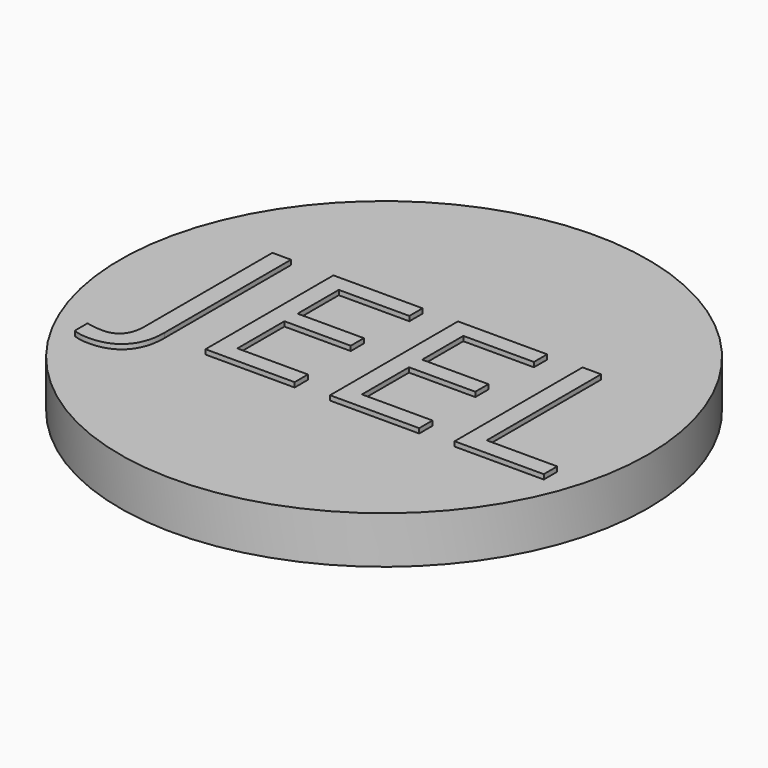
from build123d import *

# Parameters (mm, degrees)
F0_R         = 14.199997
F1_DEPTH     = 2.54
F2_TEXT_SIZE = 12.0514738632
F3_DEPTH     = 0.254


# Not quite as in the source:
# - Text() gives the source's letters only with a copy of the font that has no kerning and outlines rounded to 1/6400 em; it was checked with that copy


with BuildPart() as f1:
    # F0 (on Top) → F1 (new body)
    with BuildSketch(Plane.XY):
        Circle(F0_R)
    extrude(amount=F1_DEPTH)

    # F2 (on face) → F3 (join)
    with BuildSketch(Plane.XY.offset(2.54)):
        with Locations((-10.4060713202, -4.5045013539)):
            Text('JEEL', F2_TEXT_SIZE, font='Open Sans', text_align=(TextAlign.LEFT, TextAlign.BOTTOM))
    extrude(amount=F3_DEPTH)


solid = f1.part
